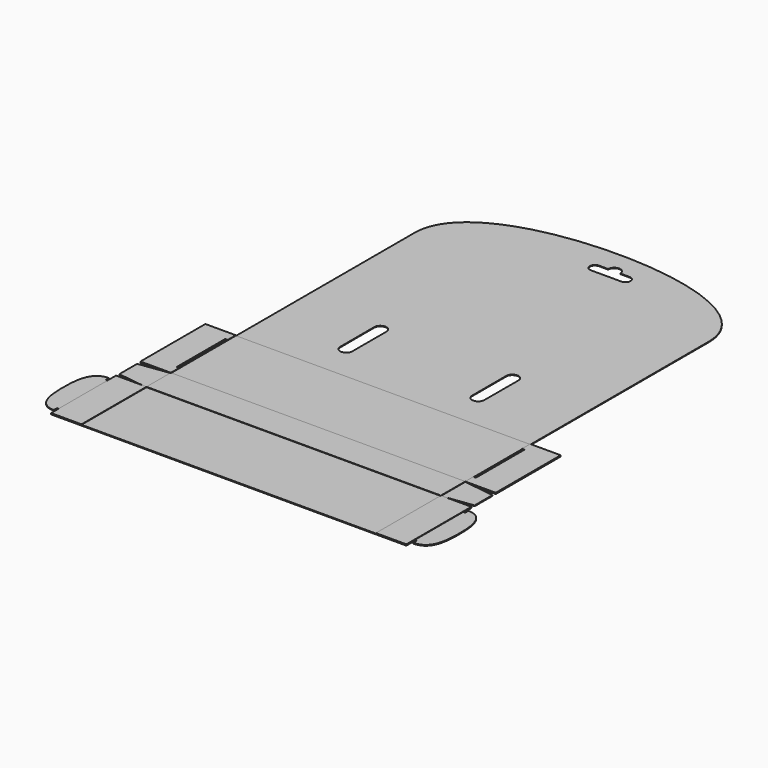
from build123d import *

# Parameters (mm, degrees)
F0_W     = 184.15
F0_H     = 50.8
F1_DEPTH = 0.508
F0_H_2   = 19.05
F2_DEPTH = 0.762
F3_DEPTH = 0.381


# Not quite as in the source:
# - ends of sketch curves that miss each other by under 0.0002 mm in the source are joined


with BuildPart() as f1:
    # F0 (on Top) → F1 (new body)
    with BuildSketch(Plane.XY):
        with Locations((92.075, 25.4)):
            Rectangle(F0_W, F0_H)
    extrude(amount=F1_DEPTH)


with BuildPart() as f1b:
    # F0 (on Top) → F1, piece 2 (new body)
    with BuildSketch(Plane.XY):
        Polygon((-19.05, 53.34), (0, 50.8), (0, 69.85), (-19.05, 67.31), align=None)
    extrude(amount=F1_DEPTH)


with BuildPart() as f1c:
    # F0 (on Top) → F1, piece 3 (new body)
    with BuildSketch(Plane.XY):
        Polygon((184.15, 69.85), (184.15, 50.8), (203.2, 53.34), (203.2, 67.31), align=None)
    extrude(amount=F1_DEPTH)


with BuildPart() as f1d:
    # F0 (on Top) → F1, piece 4 (new body)
    with BuildSketch(Plane.XY):
        Polygon((0, 76.2), (0, 69.85), (184.15, 69.85), (184.15, 76.2), (184.15, 114.3), (184.15, 120.65), (0, 120.65), (0, 114.3), align=None)
    extrude(amount=F1_DEPTH)


with BuildPart() as f1e:
    # F0 (on Top) → F1, piece 5 (new body)
    with BuildSketch(Plane.XY):
        with BuildLine():
            Line((203.2, 44.45), (203.2, 6.35))
            Line((203.2, 6.35), (204.47, 6.35))
            Line((204.47, 6.35), (204.47, 3.81))
            add(Edge.make_bspline(
                [(204.47, 46.99), (214.63, 46.762470156), (217.17, 25.5095088242), (214.63, 3.8185121957), (204.47, 3.81)],
                knots=[0, 0, 0, 0, 0.5, 1, 1, 1, 1], degree=3))
            Line((204.47, 46.99), (204.47, 44.45))
            Line((204.47, 44.45), (203.2, 44.45))
        make_face()
    extrude(amount=F1_DEPTH)


with BuildPart() as f1f:
    # F0 (on Top) → F1, piece 6 (new body)
    with BuildSketch(Plane.XY):
        with BuildLine():
            Line((-19.05, 6.35), (-19.05, 44.45))
            Line((-19.05, 44.45), (-20.32, 44.45))
            Line((-20.32, 44.45), (-20.32, 46.99))
            add(Edge.make_bspline(
                [(-20.32, 46.99), (-30.48, 46.762470156), (-33.02, 25.5095088242), (-30.48, 3.8185121957), (-20.32, 3.81)],
                knots=[0, 0, 0, 0, 0.5, 1, 1, 1, 1], degree=3))
            Line((-20.32, 3.81), (-20.32, 6.35))
            Line((-20.32, 6.35), (-19.05, 6.35))
        make_face()
    extrude(amount=F1_DEPTH)


with BuildPart() as f2:
    # F0 (on Top) → F2 (new body)
    with BuildSketch(Plane.XY):
        with Locations((92.075, 60.325)):
            Rectangle(F0_W, F0_H_2)
    extrude(amount=F2_DEPTH)


with BuildPart() as f2b:
    # F0 (on Top) → F2, piece 2 (new body)
    with BuildSketch(Plane.XY):
        Polygon((184.15, 76.2), (184.15, 69.85), (203.2, 69.85), (203.2, 120.65), (184.15, 120.65), (184.15, 114.3), (185.7375, 114.3), (185.7375, 76.2), align=None)
    extrude(amount=F2_DEPTH)


with BuildPart() as f2c:
    # F0 (on Top) → F2, piece 3 (new body)
    with BuildSketch(Plane.XY):
        Polygon((184.15, 50.8), (184.15, 0), (203.2, 0), (203.2, 6.35), (203.2, 44.45), (203.2, 50.8), align=None)
    extrude(amount=F2_DEPTH)


with BuildPart() as f2d:
    # F0 (on Top) → F2, piece 4 (new body)
    with BuildSketch(Plane.XY):
        Polygon((-19.05, 0), (0, 0), (0, 50.8), (-19.05, 50.8), (-19.05, 44.45), (-19.05, 6.35), (-19.05, 3.81), align=None)
    extrude(amount=F2_DEPTH)


with BuildPart() as f2e:
    # F0 (on Top) → F2, piece 5 (new body)
    with BuildSketch(Plane.XY):
        Polygon((-19.05, 69.85), (0, 69.85), (0, 76.2), (-1.5875, 76.2), (-1.5875, 114.3), (0, 114.3), (0, 120.65), (-19.05, 120.65), align=None)
    extrude(amount=F2_DEPTH)


with BuildPart() as f3:
    # F0 (on Top) → F3 (new body)
    with BuildSketch(Plane.XY):
        with BuildLine():
            Line((0, 260.35), (0, 120.65))
            Line((0, 120.65), (184.15, 120.65))
            Line((184.15, 120.65), (184.15, 260.35))
            add(Edge.make_bspline(
                [(0, 260.35), (0, 291.2788689137), (92.075, 318.3211310863), (184.15, 291.2788689137), (184.15, 260.35)],
                knots=[0, 0, 0, 0, 0.5, 1, 1, 1, 1], degree=3))
        make_face()
        with BuildLine():
            ThreePointArc((54.61, 143.5100303088), (53.4940670417, 140.8159436779), (50.7999722968, 139.7000303089))
            ThreePointArc((50.7999722968, 139.7000303089), (48.1088940654, 140.8129811804), (46.9900046733, 143.5015910564))
            Line((46.9900046733, 143.5015910564), (46.9309298286, 170.171560748))
            ThreePointArc((46.9309298286, 170.171560748), (48.0438819902, 172.8711119219), (50.7409783035, 173.99))
            Line((50.7409783035, 173.99), (50.8000578216, 173.9899991034))
            ThreePointArc((50.8000578216, 173.9899991034), (53.4940972793, 172.8740554971), (54.61, 170.1799991038))
            Line((54.61, 170.1799991038), (54.61, 143.5100303088))
        make_face(mode=Mode.SUBTRACT)
        with BuildLine():
            Line((129.54, 143.5100303088), (129.54, 170.1799991038))
            ThreePointArc((129.54, 170.1799991038), (130.6559027207, 172.8740554971), (133.3499421784, 173.9899991034))
            Line((133.3499421784, 173.9899991034), (133.4090216965, 173.99))
            ThreePointArc((133.4090216965, 173.99), (136.1061180098, 172.8711119219), (137.2190701714, 170.171560748))
            Line((137.2190701714, 170.171560748), (137.1599953267, 143.5015910564))
            ThreePointArc((137.1599953267, 143.5015910564), (136.0411059346, 140.8129811804), (133.3500323765, 139.7000303089))
            ThreePointArc((133.3500323765, 139.7000303089), (130.6559329583, 140.8159436779), (129.54, 143.5100303088))
        make_face(mode=Mode.SUBTRACT)
        with BuildLine():
            Line((111.125, 283.21), (92.075, 283.21))
            ThreePointArc((92.075, 283.21), (89.8299359697, 284.1399359697), (88.9, 286.385))
            ThreePointArc((88.9, 286.385), (89.8299359697, 288.6300640303), (92.075, 289.56))
            Line((92.075, 289.56), (97.79, 289.56))
            ThreePointArc((97.79, 289.56), (101.6, 293.3223531569), (105.41, 289.56))
            Line((105.41, 289.56), (111.125, 289.56))
            ThreePointArc((111.125, 289.56), (113.3700640303, 288.6300640303), (114.3, 286.385))
            ThreePointArc((114.3, 286.385), (113.3700640303, 284.1399359697), (111.125, 283.21))
        make_face(mode=Mode.SUBTRACT)
    extrude(amount=F3_DEPTH)


solid = Compound([f1.part, f1b.part, f1c.part, f1d.part, f1e.part, f1f.part, f2.part, f2b.part, f2c.part, f2d.part, f2e.part, f3.part])
